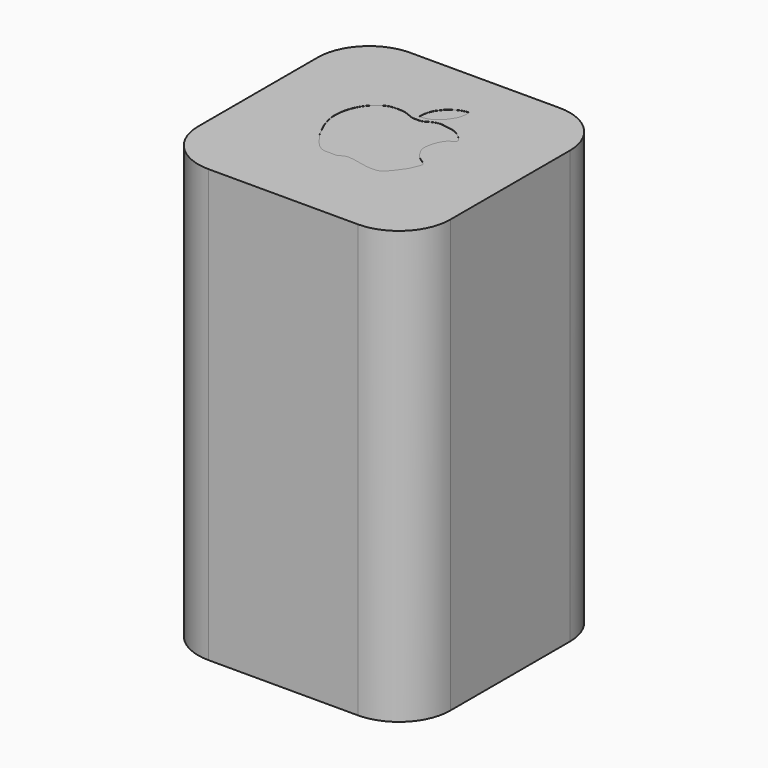
from build123d import *

# Parameters (mm, degrees)
F0_W     = 98
F0_H     = 98
F1_DEPTH = 168
F2_R     = 20
F4_DEPTH = 0.1
F5_W     = 17
F5_H     = 11
F5_H_2   = 6
F6_DEPTH = 16
F7_R     = 1.75
F8_DEPTH = 7


# Not quite as in the source:
# - a pattern or mirror of a feature is missing from the dataset's text; its kind, count and spacing are read off the source's solid


with BuildPart() as f1:
    # F0 (on Top) → F1 (new body)
    with BuildSketch(Plane.XY):
        Rectangle(F0_W, F0_H)
    extrude(amount=F1_DEPTH)

    # F2
    f2_edges = [f1.edges().sort_by_distance(p)[0] for p in [
        (-49, -49, 84),
        (49, -49, 84),
        (49, 49, 84),
        (-49, 49, 84),
    ]]
    fillet(f2_edges, radius=F2_R)

    # F3 (on face) → F4 (cut)
    with BuildSketch(Plane.XY.offset(168)):
        with BuildLine():
            add(Edge.make_bspline(
                [(-16.6899659042, 14.5263501159), (-15.7136301, 15.473474875), (-13.1302215889, 17.5396681171), (-10.163313644, 17.8625162817), (-7.8170980309, 17.8538784678), (-5.3256308293, 17.60672308), (-2.2939848942, 15.935207709), (-0.0642127732, 15.9835017091), (2.1593820078, 15.9256852578), (4.2007830475, 17.58385374), (7.2150048696, 18.4301242869), (9.4067203495, 18.005698026), (12.9413477402, 17.5124601108), (15.451449154, 16.328117072), (19.8322651108, 12.3789907506), (16.3483119576, 11.161327134), (14.9326028931, 9.2267641101), (13.8760163047, 6.9356450608), (13.2878223886, 4.2669207751), (13.116810682, 1.7047616528), (14.4278596185, -0.562625055), (16.0129662851, -3.4114646568), (20.4149124908, -5.2982240128), (19.4649996391, -7.5896092217), (18.3863623312, -10.5619664375), (16.0952905737, -13.5904763189), (13.0355533184, -17.5209757348), (10.4825747855, -17.811689469), (8.3832255666, -17.8446920455), (5.5169659138, -17.4001882307), (2.6547423027, -16.747745499), (0.4414756664, -16.255698015), (-2.3296419631, -16.2383496001), (-4.2488359517, -17.9302568959), (-6.6455336281, -17.4107400486), (-9.1173833744, -17.8743455193), (-11.8716087541, -16.4682333697), (-13.6396621681, -14.5101514655), (-15.023495226, -12.5989551886), (-17.0546757837, -10.2449876163), (-18.2749041524, -7.2461423221), (-19.6753841099, -4.868239072), (-20.6199413173, -1.7626345112), (-21.3378449337, 1.1483554628), (-21.2223337426, 3.436847423), (-20.9906414832, 6.9730961893), (-19.6659411692, 10.4008468617), (-18.3635902923, 12.631691028), (-17.4200411367, 13.8181180448), (-16.6899659042, 14.5263501159)],
                knots=[0, 0, 0, 0, 0.0269873977, 0.0486588319, 0.0676541078, 0.0876303882, 0.1108305241, 0.1296294765, 0.1477858687, 0.1680591565, 0.1899132705, 0.2089476693, 0.232055585, 0.2547145828, 0.2813540263, 0.3009602858, 0.3208345596, 0.3407430099, 0.3616626522, 0.3815025704, 0.4014110196, 0.424605639, 0.4502188675, 0.4674535269, 0.4898057779, 0.5150425906, 0.542715089, 0.5620541402, 0.5801654257, 0.601703494, 0.6233749299, 0.6425252812, 0.6629890374, 0.6823477131, 0.7013429878, 0.721182906, 0.7428543404, 0.7632871479, 0.7826261908, 0.8048078965, 0.8274668939, 0.8484450584, 0.8712187942, 0.8928902303, 0.9118855012, 0.9355810169, 0.9598985807, 0.9798196168, 1, 1, 1, 1], degree=3))
        make_face()
        with BuildLine():
            add(Edge.make_bspline(
                [(9.2462628775, 29.4047111104), (9.4489872186, 29.2359268152), (9.5475627918, 28.3150921555), (9.591111392, 27.2079295375), (9.2361191197, 25.9047900362), (8.9285869111, 24.5821274214), (8.179025351, 23.4884265558), (7.4347156368, 22.421243903), (6.8102353155, 21.4270992504), (5.8755987486, 20.5567472454), (5.0186611953, 19.8074004567), (4.2366087758, 19.2143237784), (2.7247127642, 18.4849628882), (1.1527423174, 17.9962101021), (0.1977089178, 18.0766353228), (-0.7729787247, 17.8464430875), (-0.6341887473, 18.6485781673), (-0.7232774473, 19.5492995182), (-0.5163363199, 20.6775121148), (-0.2433638059, 21.7479778158), (0.162811632, 22.8022604986), (0.6280750732, 23.9246849059), (1.3213365269, 24.6495548656), (2.0913898878, 25.7663970648), (2.859092629, 26.7584245726), (4.2122840025, 27.5241985904), (5.105289444, 28.2653268578), (6.6317880587, 29.0321734979), (8.3115327411, 29.3784917144), (9.0646087688, 29.555952745), (9.2462628775, 29.4047111104)],
                knots=[0, 0, 0, 0, 0.0335563199, 0.0691340182, 0.1067996851, 0.1448667939, 0.1823613199, 0.2196122447, 0.2550274639, 0.2919580032, 0.3265473354, 0.358749939, 0.4012497625, 0.4431452283, 0.4761091527, 0.504101529, 0.5287136161, 0.5607241268, 0.5956380721, 0.6300504612, 0.6649857196, 0.7005835708, 0.7333427469, 0.7710592834, 0.8080258226, 0.8480875453, 0.8835027825, 0.926002606, 0.9699313691, 1, 1, 1, 1], degree=3))
        make_face()
    extrude(amount=-F4_DEPTH, mode=Mode.SUBTRACT)

    # F5 (on face) → F6 (cut)
    with BuildSketch(Plane(origin=(0, 49, 0), x_dir=(-1, 0, 0), z_dir=(0, 1, 0))):
        with BuildLine():
            Line((-4, 9), (4, 9))
            ThreePointArc((4, 9), (10, 15), (4, 21))
            Line((4, 21), (-4, 21))
            ThreePointArc((-4, 21), (-10, 15), (-4, 9))
        make_face()
        with Locations((0, 30.5)):
            Rectangle(F5_W, F5_H)
        with Locations((0, 44)):
            Rectangle(F5_W, F5_H_2)
        with Locations((0, 57.5)):
            Rectangle(F5_W, F5_H)
        with Locations((0, 73.5)):
            Rectangle(F5_W, F5_H)
        with Locations((0, 89.5)):
            Rectangle(F5_W, F5_H)
    extrude(amount=-F6_DEPTH, mode=Mode.SUBTRACT)

    # F7 (on face) → F8 (join)
    with BuildSketch(Plane(origin=(0, 33, 0), x_dir=(-1, 0, 0), z_dir=(0, 1, 0))):
        with Locations((4, 15)):
            Circle(F7_R)
    f8 = extrude(amount=F8_DEPTH)

    # F8_copies: F8 across plane
    add(f8.mirror(Plane(origin=(0, 0, 0), x_dir=(0, 0, 1), z_dir=(1, 0, 0))))


solid = f1.part
